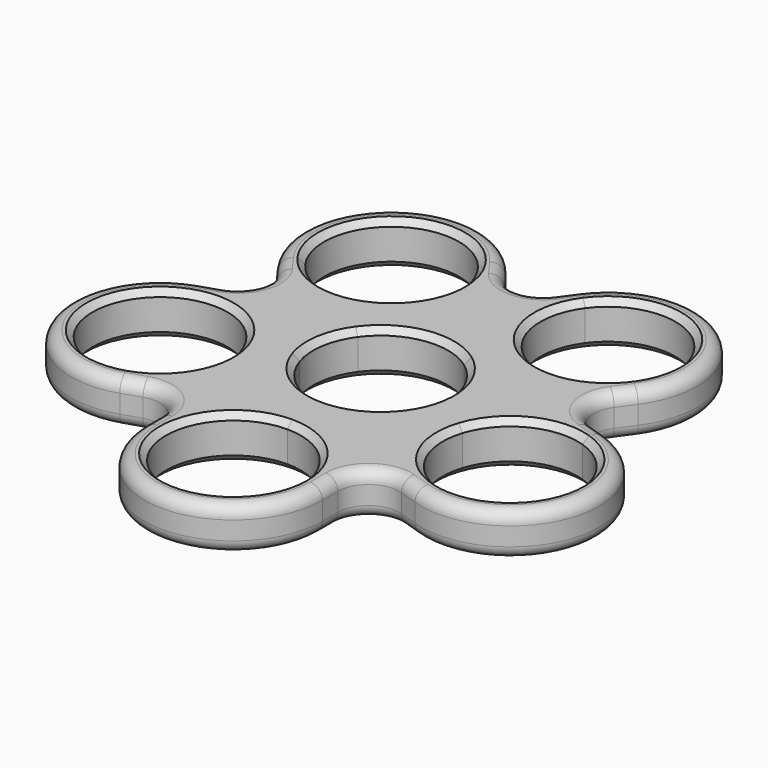
from build123d import *

# Parameters (mm, degrees)
F1_DEPTH = 7
F3_DEPTH = 7.001
F5_COUNT = 5
F7_R     = 5
F8_R     = 2
F9_SIZE  = 1


# Not quite as in the source:
# - a feature names something its author has since deleted; it is built from what else it names


with BuildPart() as f1:
    # F0 (on Top) → F1 (new body)
    with BuildSketch(Plane.XY):
        with BuildLine():
            ThreePointArc((-14.5, 0), (0, -14.5), (14.5, 0))
            ThreePointArc((14.5, 0), (0, 14.5), (-14.5, 0))
        make_face()
        with BuildLine():
            Line((14.5, -30), (14.5, 0))
            ThreePointArc((14.5, 0), (0, -14.5), (-14.5, 0))
            Line((-14.5, 0), (-14.5, -30))
            ThreePointArc((-14.5, -30), (0, -15.5), (14.5, -30))
        make_face()
        with BuildLine():
            ThreePointArc((-14.5, -30), (0, -44.5), (14.5, -30))
            ThreePointArc((14.5, -30), (0, -15.5), (-14.5, -30))
        make_face()
    extrude(amount=F1_DEPTH)

    # F2 (on face) → F3 (cut, through all)
    with BuildSketch(Plane.XY.offset(7)):
        with BuildLine():
            ThreePointArc((0, -11), (7.7781745931, -7.7781745931), (11, 0))
            ThreePointArc((11, 0), (-7.7781745931, 7.7781745931), (0, -11))
        make_face()
        with BuildLine():
            ThreePointArc((11, -30), (7.7781745931, -22.2218254069), (0, -19))
            ThreePointArc((0, -19), (-7.7781745931, -37.7781745931), (11, -30))
        make_face()
    extrude(amount=-F3_DEPTH, mode=Mode.SUBTRACT)


with BuildPart() as f5_1:
    # F5: instance of F1
    add(f1.part.rotate(Axis((0, 0, 13.2415927947), (0, 0, 1)), 1 * 360 / F5_COUNT))


with BuildPart() as f5_2:
    # F5: instance of F1
    add(f1.part.rotate(Axis((0, 0, 13.2415927947), (0, 0, 1)), 2 * 360 / F5_COUNT))


with BuildPart() as f5_3:
    # F5: instance of F1
    add(f1.part.rotate(Axis((0, 0, 13.2415927947), (0, 0, 1)), 3 * 360 / F5_COUNT))


with BuildPart() as f5_4:
    # F5: instance of F1
    add(f1.part.rotate(Axis((0, 0, 13.2415927947), (0, 0, 1)), 4 * 360 / F5_COUNT))

    # F6: union F5_3, F5_2, F5_1, F1
    add(f5_3.part)
    add(f5_2.part)
    add(f5_1.part)
    add(f1.part)

    # F7
    f7_edges = [f5_4.edges().sort_by_distance(p)[0] for p in [
        (-14.5, -19.957538, 3.5),
        (14.5, -19.957538, 3.5),
        (23.461493, 7.623101, 3.5),
        (-23.461493, 7.623101, 3.5),
        (0, 24.668873, 3.5),
    ]]
    fillet(f7_edges, radius=F7_R)

    # F8
    f8_edges = [f5_4.edges().sort_by_distance(p)[0] for p in [
        (42.322015, -13.751256, 7),
        (0, -44.5, 0),
        (14.5, -28.419724, 0),
        (16.561074, -22.794362, 0),
        (22.548017, -22.572497, 0),
        (-14.5, -28.419724, 0),
        (42.322015, -13.751256, 0),
        (-16.561074, -22.794362, 0),
        (31.50951, 5.008142, 0),
        (-22.548017, -22.572497, 0),
        (26.79638, 8.706672, 0),
        (-42.322015, -13.751256, 0),
        (28.435441, 14.469153, 0),
        (-31.50951, 5.008142, 0),
        (26.156444, 36.001256, 0),
        (-26.79638, 8.706672, 0),
        (4.973948, 31.514926, 0),
        (-28.435441, 14.469153, 0),
        (0, 28.175382, 0),
        (-26.156444, 36.001256, 0),
        (-4.973948, 31.514926, 0),
        (14.5, -28.419724, 7),
        (16.561074, -22.794362, 7),
        (0, -44.5, 7),
        (22.548017, -22.572497, 7),
        (-14.5, -28.419724, 7),
        (-16.561074, -22.794362, 7),
        (31.50951, 5.008142, 7),
        (-22.548017, -22.572497, 7),
        (26.79638, 8.706672, 7),
        (-42.322015, -13.751256, 7),
        (28.435441, 14.469153, 7),
        (-31.50951, 5.008142, 7),
        (26.156444, 36.001256, 7),
        (-26.79638, 8.706672, 7),
        (4.973948, 31.514926, 7),
        (-28.435441, 14.469153, 7),
        (0, 28.175382, 7),
        (-26.156444, 36.001256, 7),
        (-4.973948, 31.514926, 7),
    ]]
    fillet(f8_edges, radius=F8_R)

    # F9
    f9_edges = [f5_4.edges().sort_by_distance(p)[0] for p in [
        (10.461622, 3.399187, 7),
        (24.099195, 33.169697, 7),
        (-24.099195, 33.169697, 7),
        (-38.993317, -12.669697, 7),
        (0, -41, 7),
        (38.993317, -12.669697, 7),
        (0, -41, 0),
        (38.993317, -12.669697, 0),
        (24.099195, 33.169697, 0),
        (-24.099195, 33.169697, 0),
        (10.461622, 3.399187, 0),
        (-38.993317, -12.669697, 0),
    ]]
    chamfer(f9_edges, length=F9_SIZE)


solid = f5_4.part
